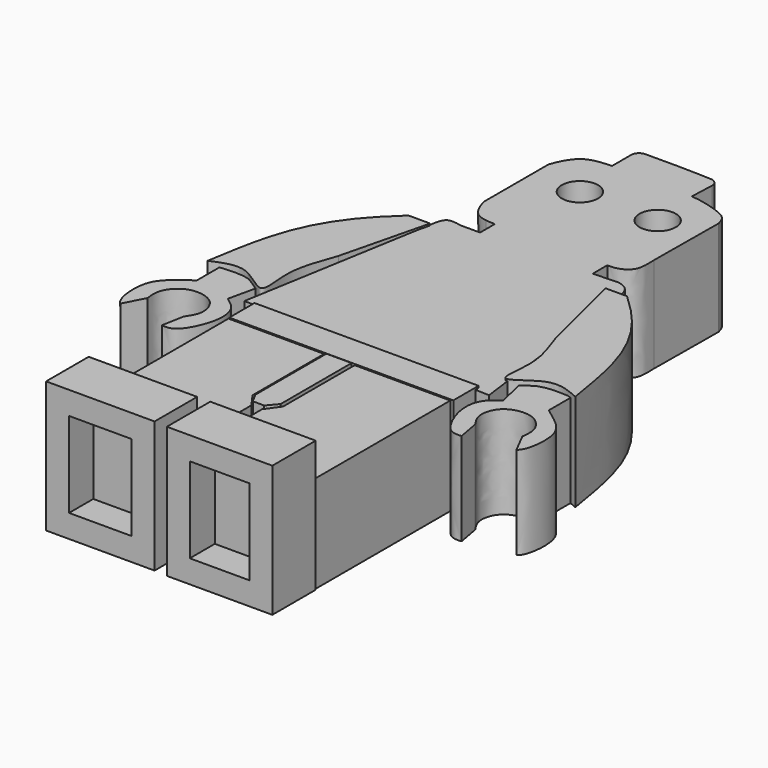
from build123d import *

# Parameters (mm, degrees)
F6_DEPTH  = 10.4
F7_DEPTH  = 10.6
F8_DEPTH  = 10.6
F9_DEPTH  = 10.7
F5_W      = 11.8155628443
F5_H      = 5.798378028
F10_DEPTH = 14.3
F5_W_2    = 11.4873507991
F5_H_2    = 5.9077814221
F12_DEPTH = 10.1
F11_W     = 24.3986994028
F11_H     = 3.4365914762
F13_DEPTH = 10.6
F14_T     = -2.5
F15_T     = -2.5
F16_R     = 1.9762807691
F17_DEPTH = 2.3


with BuildPart() as f6:
    # F0 (on Top) → F6 (new body)
    with BuildSketch(Plane.XY):
        with BuildLine():
            Line((-32.0325870551, 66.7641535401), (-32.0325870551, 58.0471716821))
            add(Edge.make_bspline(
                [(-32.0325870551, 58.0471716821), (-31.8269497763, 57.1503502742), (-31.2687347143, 55.818909493), (-30.1766841991, 55.4862767769), (-29.7736380455, 55.4269208871)],
                knots=[0, 0, 0, 0, 0.5182766208, 0.7834445384, 0.7834445384, 0.7834445384, 0.7834445384], degree=3))
            add(Edge.make_bspline(
                [(-29.7736380455, 55.4269208871), (-29.4444811601, 55.3784465384), (-29.0930305372, 55.3654731014), (-28.7343896925, 55.3546696901)],
                knots=[0.7834445384, 0.7834445384, 0.7834445384, 0.7834445384, 1, 1, 1, 1], degree=3))
            Line((-28.7343896925, 55.3546696901), (-28.7343896925, 53.3520914614))
            Line((-28.7343896925, 53.3520914614), (-30.8547690511, 53.3520914614))
            add(Edge.make_bspline(
                [(-30.8547690511, 53.3520914614), (-31.444275706, 53.4790789924), (-32.6839152606, 53.7461137493), (-32.8749563197, 52.3285525256), (-32.9751484096, 51.5851080418)],
                knots=[0, 0, 0, 0, 0.4755468255, 1, 1, 1, 1], degree=3))
            Line((-32.9751484096, 51.5851080418), (-36.5091115236, 30.9703145176))
            Line((-36.5091115236, 30.9703145176), (-22.9622479528, 30.9703145176))
            Line((-22.9622479528, 30.9703145176), (-9.4258561429, 30.4377646382))
            Line((-9.4258561429, 30.4377646382), (-12.1466854591, 51.1755488777))
            add(Edge.make_bspline(
                [(-14.3740310411, 53.5048191972), (-13.7554949673, 53.612810346), (-12.3313214707, 53.1584017832), (-12.2149238007, 51.8944370891), (-12.1466854591, 51.1755488777)],
                knots=[0, 0, 0, 0, 0.4951541185, 1, 1, 1, 1], degree=3))
            Line((-14.3740310411, 53.5048191972), (-16.5244787931, 53.4245419758))
            Line((-16.5244787931, 53.4245419758), (-16.5244787931, 55.4202012718))
            add(Edge.make_bspline(
                [(-16.5244787931, 55.4202012718), (-15.7584742986, 55.3067191244), (-13.7779941454, 55.9328043038), (-14.0099802776, 57.7935097155), (-14.015994966, 58.6299821734)],
                knots=[0, 0, 0, 0, 0.4951349422, 1, 1, 1, 1], degree=3))
            Line((-14.015994966, 58.6299821734), (-13.944814157, 67.3466715457))
            add(Edge.make_bspline(
                [(-13.944814157, 67.3466715457), (-14.1805967589, 68.1569556164), (-14.6378384853, 68.8902116144), (-17.5641442448, 69.7058372132), (-18.8332136804, 69.8016632883)],
                knots=[0, 0, 0, 0, 0.3937873539, 1, 1, 1, 1], degree=3))
            Line((-18.8332136804, 69.8016632883), (-18.7306558446, 72.4084858626))
            ThreePointArc((-18.7306558446, 72.4084858626), (-18.9593469007, 73.0284791815), (-19.5594573773, 73.305171665))
            Line((-19.5594573773, 73.305171665), (-20.9408988765, 73.3595204541))
            Line((-20.9408988765, 73.3595204541), (-23.3156438917, 73.4062161025))
            Line((-23.3156438917, 73.4062161025), (-26.7733832868, 73.4062161025))
            ThreePointArc((-26.7733832868, 73.4062161025), (-27.3839071211, 73.1533288502), (-27.6367943734, 72.5428050159))
            Line((-27.6367943734, 72.5428050159), (-27.6367943734, 69.9339658022))
            add(Edge.make_bspline(
                [(-32.0325870551, 66.7641535401), (-31.6870094182, 67.7983368992), (-30.696980441, 69.7949859621), (-28.6673216468, 69.8968052742), (-27.6367943734, 69.9339658022)],
                knots=[0, 0, 0, 0, 0.5088131843, 1, 1, 1, 1], degree=3))
        make_face()
    extrude(amount=F6_DEPTH)

    # F1 (on Top) → F7 (join)
    with BuildSketch(Plane.XY):
        with BuildLine():
            Line((-35.2133251727, 42.1612039208), (-32.8573472798, 51.7029054463))
            Line((-32.8573472798, 51.7029054463), (-35.2133251727, 51.7029054463))
            add(Edge.make_bspline(
                [(-35.2133251727, 51.7029054463), (-36.2951818867, 50.6858613868), (-38.6379629922, 48.4834333062), (-41.9718158913, 42.9838888747), (-42.8602654205, 37.4833367687), (-43.3414429426, 34.5042794943)],
                knots=[0, 0, 0, 0, 0.2822834697, 0.6112901743, 1, 1, 1, 1], degree=3))
            add(Edge.make_bspline(
                [(-35.2133251727, 42.1612039208), (-35.6208050014, 41.0260900753), (-36.404568041, 38.8427665953), (-36.6687184167, 36.2694539944), (-35.9728910598, 32.0898037392), (-39.8262291077, 36.0696283167), (-42.157769761, 35.0313772778), (-43.3414429426, 34.5042794943)],
                knots=[0, 0, 0, 0, 0.2081509016, 0.4003657895, 0.5763524651, 0.7849232332, 1, 1, 1, 1], degree=3))
        make_face()
        with BuildLine():
            Line((-11.4179626107, 51.7029054463), (-13.7739405036, 51.7029054463))
            Line((-13.7739405036, 51.7029054463), (-11.4179626107, 42.1612039208))
            add(Edge.make_bspline(
                [(-11.4179626107, 42.1612039208), (-11.010482782, 41.0260900753), (-10.2267197424, 38.8427665953), (-9.9625693666, 36.2694539944), (-10.6583967236, 32.0898037392), (-6.8050586757, 36.0696283167), (-4.4735180224, 35.0313772778), (-3.2898448408, 34.5042794943)],
                knots=[0, 0, 0, 0, 0.2081509016, 0.4003657895, 0.5763524651, 0.7849232332, 1, 1, 1, 1], degree=3))
            add(Edge.make_bspline(
                [(-11.4179626107, 51.7029054463), (-10.3361058967, 50.6858613868), (-7.9933247912, 48.4834333062), (-4.659471892, 42.9838888747), (-3.7710223629, 37.4833367687), (-3.2898448408, 34.5042794943)],
                knots=[0, 0, 0, 0, 0.2822834697, 0.6112901743, 1, 1, 1, 1], degree=3))
        make_face()
    extrude(amount=F7_DEPTH)

    # F2 (on Top) → F12 (join)
    with BuildSketch(Plane.XY):
        with BuildLine():
            add(Edge.make_bspline(
                [(-42.3993654549, 34.9732488394), (-41.5083657131, 35.0395030605), (-39.7607124628, 35.169457537), (-38.2334864364, 34.5347135996), (-37.4848805368, 34.2235788703)],
                knots=[0, 0, 0, 0, 0.5098263867, 1, 1, 1, 1], degree=3))
            Line((-42.3993654549, 34.9732488394), (-42.3993654549, 31.8912826478))
            add(Edge.make_bspline(
                [(-42.3993654549, 31.8912826478), (-42.8214044408, 31.5822794047), (-43.777415733, 30.8823189753), (-45.9351517853, 29.0997607374), (-45.5344700245, 25.262844347), (-44.9557346096, 24.6141590411), (-44.7996284019, 24.4847049468)],
                knots=[0, 0, 0, 0, 0.2201722589, 0.4987386777, 0.8291601062, 0.9435640578, 0.9435640578, 0.9435640578, 0.9435640578], degree=3))
            Line((-44.7996284019, 24.4847049468), (-43.6488091946, 26.7269108444))
            add(Edge.make_bspline(
                [(-43.6488091946, 26.7269108444), (-43.7087373386, 27.2334529886), (-43.829964053, 28.258120795), (-42.8972684916, 29.6874583348), (-41.3501797011, 30.4600671196), (-38.8678357555, 29.8890620575), (-38.0966588507, 27.494839303), (-38.7912331215, 26.4655003975), (-39.120698185, 25.977242738)],
                knots=[0, 0, 0, 0, 0.152205785, 0.3078921856, 0.467360414, 0.6544729412, 0.8361023448, 1, 1, 1, 1], degree=3))
            Line((-39.120698185, 25.977242738), (-39.5672880113, 23.5616490245))
            add(Edge.make_bspline(
                [(-38.2345467806, 30.8917276561), (-37.7311404598, 30.530232188), (-36.6363682172, 29.7440775687), (-36.2132651178, 27.1492758169), (-37.9338986283, 23.4240136846), (-39.120698185, 23.5240177388), (-39.5672880113, 23.5616490245)],
                knots=[0, 0, 0, 0, 0.2240020503, 0.4871437184, 0.8070134114, 1, 1, 1, 1], degree=3))
            Line((-38.2345467806, 30.8917276561), (-37.4848805368, 34.2235788703))
        make_face()
        with BuildLine():
            add(Edge.make_bspline(
                [(-8.2478672266, 30.8917276561), (-8.7512735473, 30.530232188), (-9.84604579, 29.7440775687), (-10.2691488894, 27.1492758169), (-8.5485153788, 23.4240136846), (-7.3617158222, 23.5240177388), (-6.9151259959, 23.5616490245)],
                knots=[0, 0, 0, 0, 0.2240020503, 0.4871437184, 0.8070134114, 1, 1, 1, 1], degree=3))
            Line((-6.9151259959, 23.5616490245), (-7.3617158222, 25.977242738))
            add(Edge.make_bspline(
                [(-2.8336048126, 26.7269108444), (-2.7736766686, 27.2334529886), (-2.6524499542, 28.258120795), (-3.5851455156, 29.6874583348), (-5.1322343061, 30.4600671196), (-7.6145782517, 29.8890620575), (-8.3857551565, 27.494839303), (-7.6911808856, 26.4655003975), (-7.3617158222, 25.977242738)],
                knots=[0, 0, 0, 0, 0.152205785, 0.3078921856, 0.467360414, 0.6544729412, 0.8361023448, 1, 1, 1, 1], degree=3))
            Line((-2.8336048126, 26.7269108444), (-1.6827856053, 24.4847049468))
            add(Edge.make_bspline(
                [(-4.0830485523, 31.8912826478), (-3.6610095664, 31.5822794047), (-2.7049982742, 30.8823189753), (-0.5472622219, 29.0997607374), (-0.9479439827, 25.262844347), (-1.5266793976, 24.6141590411), (-1.6827856053, 24.4847049468)],
                knots=[0, 0, 0, 0, 0.2201722589, 0.4987386777, 0.8291601062, 0.9435640578, 0.9435640578, 0.9435640578, 0.9435640578], degree=3))
            Line((-4.0830485523, 31.8912826478), (-4.0830485523, 34.9732488394))
            add(Edge.make_bspline(
                [(-4.0830485523, 34.9732488394), (-4.9740482941, 35.0395030605), (-6.7217015444, 35.169457537), (-8.2489275708, 34.5347135996), (-8.9975334704, 34.2235788703)],
                knots=[0, 0, 0, 0, 0.5098263867, 1, 1, 1, 1], degree=3))
            Line((-8.9975334704, 34.2235788703), (-8.2478672266, 30.8917276561))
        make_face()
    extrude(amount=F12_DEPTH)

    # F11 (on Top) → F13 (join)
    with BuildSketch(Plane.XY):
        with Locations((-23.1681093574, 29.2180236429)):
            Rectangle(F11_W, F11_H)
    extrude(amount=F13_DEPTH)

    # F16 (on face) → F17 (cut)
    with BuildSketch(Plane.XY.offset(10.4)):
        with Locations((-26.7982557416, 64.5196586847)):
            Circle(F16_R)
        with Locations((-18.330078572, 64.5196586847)):
            Circle(F16_R)
    extrude(amount=-F17_DEPTH, mode=Mode.SUBTRACT)


with BuildPart() as f8:
    # F3 (on Top) → F8 (new body)
    with BuildSketch(Plane.XY):
        Polygon((-35.3035181761, 27.3088160902), (-35.3035181761, 8.4005445242), (-23.8086208701, 8.4005445242), (-23.8086208701, 16.0638093948), (-24.8914733529, 17.5631437451), (-24.8914733529, 27.3088160902), align=None)
    extrude(amount=F8_DEPTH)


with BuildPart() as f8b:
    # F3 (on Top) → F8, piece 2 (new body)
    with BuildSketch(Plane.XY):
        Polygon((-21.5596184134, 17.5631437451), (-22.6424708962, 16.0638093948), (-22.6424708962, 8.4005445242), (-11.1475735903, 8.4005445242), (-11.1475735903, 27.3088160902), (-21.5596184134, 27.3088160902), align=None)
    extrude(amount=F8_DEPTH)


with BuildPart() as f9:
    # F4 (on Top) → F9 (new body)
    with BuildSketch(Plane.XY):
        Polygon((-21.8928046525, 27.3088160902), (-24.641584605, 27.3088160902), (-24.641584605, 17.6464393735), (-24.058509618, 16.5635868907), (-22.8090658784, 16.5635868907), (-21.8928046525, 17.6464393735), align=None)
    extrude(amount=F9_DEPTH)


with BuildPart() as f10:
    # F5 (on Top) → F10 (new body)
    with BuildSketch(Plane.XY):
        with Locations((-29.8467688262, 5.9463963844)):
            Rectangle(F5_W, F5_H)
    extrude(amount=F10_DEPTH)

    # F14
    f14_openings = [f10.faces().sort_by_distance(p)[0] for p in [
        (-29.846769, 3.047207, 7.15),
    ]]
    offset(amount=F14_T, openings=f14_openings)


with BuildPart() as f10b:
    # F5 (on Top) → F10, piece 2 (new body)
    with BuildSketch(Plane.XY):
        with Locations((-16.7730688117, 5.8916946873)):
            Rectangle(F5_W_2, F5_H_2)
    extrude(amount=F10_DEPTH)

    # F15
    f15_openings = [f10b.faces().sort_by_distance(p)[0] for p in [
        (-16.773069, 2.937804, 7.15),
    ]]
    offset(amount=F15_T, openings=f15_openings)


solid = Compound([f6.part, f8.part, f8b.part, f9.part, f10.part, f10b.part])
